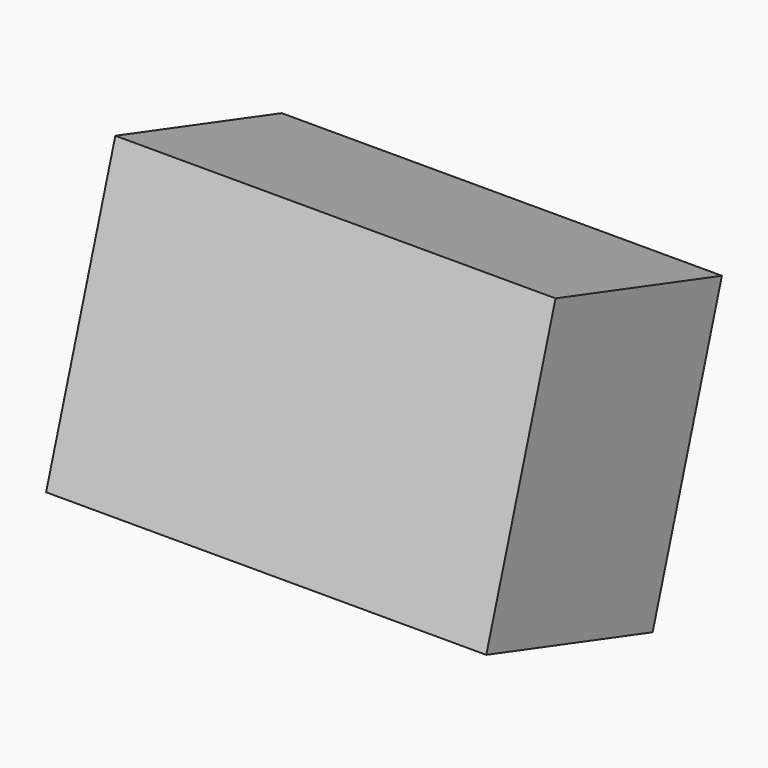
from build123d import *

# Parameters (mm, degrees)
F1_E1_W  = 88.3412
F1_E1_H  = 178.562
F2_DEPTH = 118.364


with BuildPart() as f2:
    # F1_E1 (on explicit) → F2 (new body)
    with BuildSketch(Plane(origin=(0, 36.5737514276, -50.3533995333), x_dir=(0, -0.9549597831, 0.2967352568), z_dir=(0, -0.2967352568, -0.9549597831))):
        with Locations((44.1706, 89.281)):
            Rectangle(F1_E1_W, F1_E1_H)
    extrude(amount=-F2_DEPTH)


solid = f2.part
